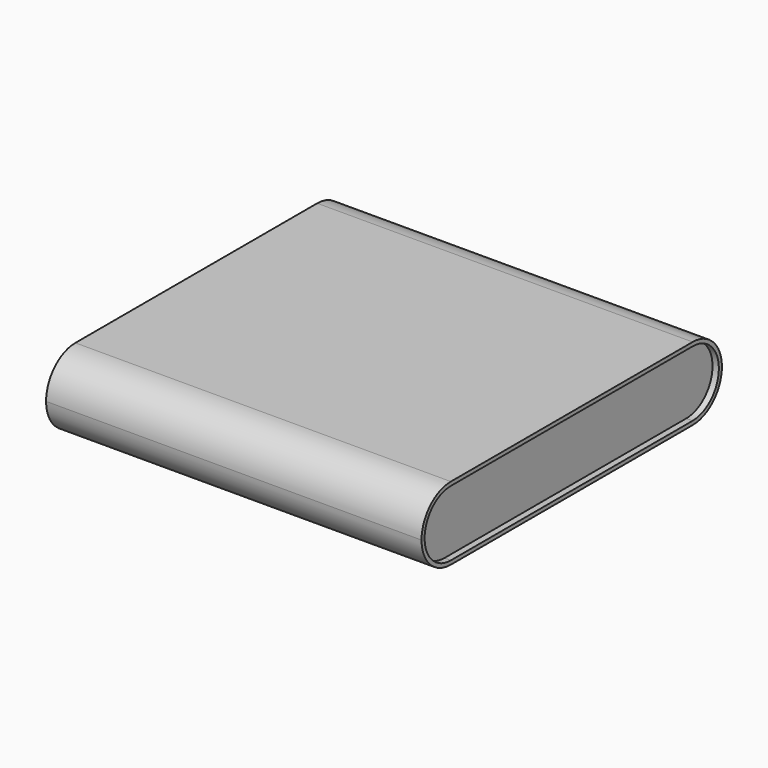
from build123d import *

# Parameters (mm, degrees)
F0_W     = 59
F0_H     = 59
F1_DEPTH = 11.5
F2_R     = 5.74999
F4_DEPTH = 1
F6_DEPTH = 1


# Not quite as in the source:
# - a fillet or chamfer is up to 0.001 mm smaller than in the source, because OpenCascade refuses the exact size


with BuildPart() as f1:
    # F0 (on Top) → F1 (new body)
    with BuildSketch(Plane.XY):
        with Locations((29.5, -29.5)):
            Rectangle(F0_W, F0_H)
    extrude(amount=F1_DEPTH)

    # F2 (radius 5.75 in the source; OpenCascade refuses exactly that, so slightly less here)
    f2_edges = [f1.edges().sort_by_distance(p)[0] for p in [
        (29.5, -59, 11.5),
        (29.5, -59, 0),
        (29.5, 0, 11.5),
        (29.5, 0, 0),
    ]]
    fillet(f2_edges, radius=F2_R)

    # F3 (on face) → F4 (cut)
    with BuildSketch(Plane.YZ.offset(59)):
        with BuildLine():
            ThreePointArc((-5.75, 0.5999998897), (-0.5999998897, 5.75), (-5.75, 10.9000001103))
            Line((-5.75, 10.9000001103), (-53.25, 10.9000001103))
            ThreePointArc((-53.25, 10.9000001103), (-58.4000001103, 5.75), (-53.25, 0.5999998897))
            Line((-53.25, 0.5999998897), (-5.75, 0.5999998897))
        make_face()
    extrude(amount=-F4_DEPTH, mode=Mode.SUBTRACT)

    # F5 (on face) → F6 (cut)
    with BuildSketch(Plane(origin=(0, 0, 0), x_dir=(0, -1, 0), z_dir=(-1, 0, 0))):
        with BuildLine():
            Line((53.25, 10.9), (5.75, 10.9))
            ThreePointArc((5.75, 10.9), (0.6, 5.75), (5.75, 0.6))
            Line((5.75, 0.6), (53.25, 0.6))
            ThreePointArc((53.25, 0.6), (58.4, 5.75), (53.25, 10.9))
        make_face()
    extrude(amount=-F6_DEPTH, mode=Mode.SUBTRACT)


solid = f1.part
